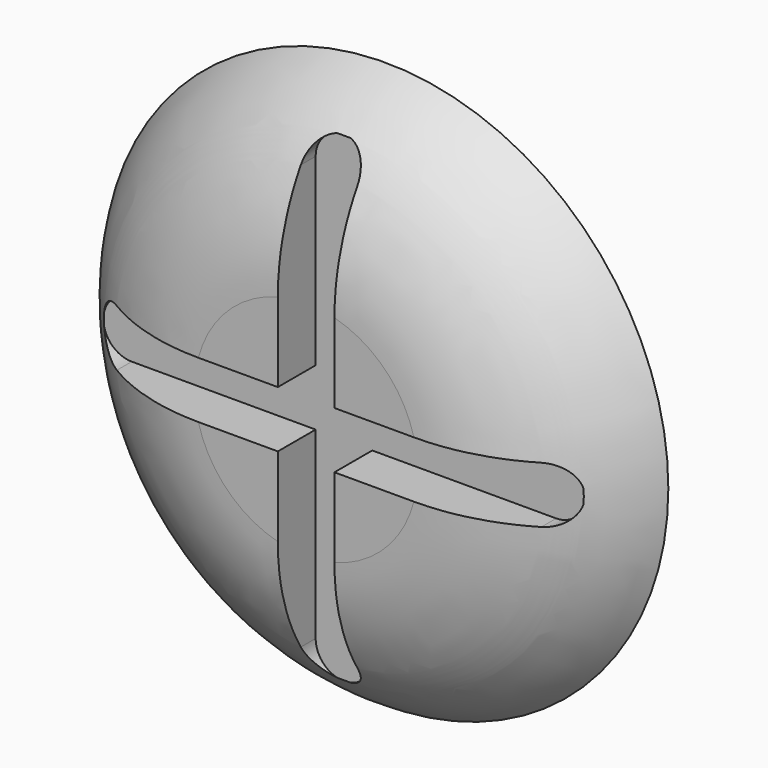
from build123d import *

# Parameters (mm, degrees)
F0_R     = 25.4
F1_DEPTH = 8.89
F3_W     = 5.08
F3_H     = 5.08
F4_DEPTH = 4.2418


# Not quite as in the source:
# - a fillet or chamfer that OpenCascade refuses, or shapes differently, is made with other operations: its cross-section is extruded or revolved along the edge and cut away or added


with BuildPart() as f1:
    # F0 (on Front) → F1 (new body)
    with BuildSketch(Plane.XZ):
        Circle(F0_R)
    extrude(amount=F1_DEPTH)

    # F2: fillet of radius 17.7830971004 on 1 edges, made by hand

    # F2_s1 → F2_t2 (revolve, cut)
    with BuildSketch(Plane.XY):
        with BuildLine():
            ThreePointArc((25.4, 0), (18.8910545541, -6.507963768), (10.0002803128, -8.89))
            Line((10.0002803128, -8.89), (25.4, -8.89))
            Line((25.4, -8.89), (25.4, 0))
        make_face()
    revolve(axis=Axis((0, -8.89, 0), (0, -1, 0)), mode=Mode.SUBTRACT)

    # F3 (on face) → F4 (cut)
    with BuildSketch(Plane.XZ.offset(8.89)):
        with BuildLine():
            Line((2.54, 19.05), (-2.54, 19.05))
            Line((-2.54, 19.05), (-2.54, 9.6723320008))
            ThreePointArc((-2.54, 9.6723320008), (0, 10.0002803128), (2.54, 9.6723320008))
            Line((2.54, 9.6723320008), (2.54, 19.05))
        make_face()
        with BuildLine():
            ThreePointArc((2.54, 19.05), (0, 21.59), (-2.54, 19.05))
            Line((-2.54, 19.05), (2.54, 19.05))
        make_face()
        with BuildLine():
            ThreePointArc((2.54, 9.6723320008), (0, 10.0002803128), (-2.54, 9.6723320008))
            Line((-2.54, 9.6723320008), (-2.54, 2.54))
            Line((-2.54, 2.54), (2.54, 2.54))
            Line((2.54, 2.54), (2.54, 9.6723320008))
        make_face()
        Rectangle(F3_W, F3_H)
        with BuildLine():
            Line((2.54, -2.54), (-2.54, -2.54))
            Line((-2.54, -2.54), (-2.54, -9.6723320008))
            ThreePointArc((-2.54, -9.6723320008), (0, -10.0002803128), (2.54, -9.6723320008))
            Line((2.54, -9.6723320008), (2.54, -2.54))
        make_face()
        with BuildLine():
            Line((2.54, -19.05), (-2.54, -19.05))
            ThreePointArc((-2.54, -19.05), (0, -21.59), (2.54, -19.05))
        make_face()
        with BuildLine():
            ThreePointArc((2.54, -9.6723320008), (0, -10.0002803128), (-2.54, -9.6723320008))
            Line((-2.54, -9.6723320008), (-2.54, -19.05))
            Line((-2.54, -19.05), (2.54, -19.05))
            Line((2.54, -19.05), (2.54, -9.6723320008))
        make_face()
        with BuildLine():
            Line((9.6723320008, 2.54), (2.54, 2.54))
            Line((2.54, 2.54), (2.54, -2.54))
            Line((2.54, -2.54), (9.6723320008, -2.54))
            ThreePointArc((9.6723320008, -2.54), (9.9179543662, -1.2805418868), (10.0002803128, 0))
            ThreePointArc((10.0002803128, 0), (9.9179543662, 1.2805418868), (9.6723320008, 2.54))
        make_face()
        with BuildLine():
            Line((19.05, 2.54), (9.6723320008, 2.54))
            ThreePointArc((9.6723320008, 2.54), (9.9179543662, 1.2805418868), (10.0002803128, 0))
            ThreePointArc((10.0002803128, 0), (9.9179543662, -1.2805418868), (9.6723320008, -2.54))
            Line((9.6723320008, -2.54), (19.05, -2.54))
            Line((19.05, -2.54), (19.05, 2.54))
        make_face()
        with BuildLine():
            ThreePointArc((19.05, -2.54), (21.59, 0), (19.05, 2.54))
            Line((19.05, 2.54), (19.05, -2.54))
        make_face()
        with BuildLine():
            Line((-2.54, -2.54), (-2.54, 2.54))
            Line((-2.54, 2.54), (-9.6723320008, 2.54))
            ThreePointArc((-9.6723320008, 2.54), (-10.0002803128, 0), (-9.6723320008, -2.54))
            Line((-9.6723320008, -2.54), (-2.54, -2.54))
        make_face()
        with BuildLine():
            ThreePointArc((-9.6723320008, -2.54), (-10.0002803128, 0), (-9.6723320008, 2.54))
            Line((-9.6723320008, 2.54), (-19.05, 2.54))
            Line((-19.05, 2.54), (-19.05, -2.54))
            Line((-19.05, -2.54), (-9.6723320008, -2.54))
        make_face()
        with BuildLine():
            Line((-19.05, -2.54), (-19.05, 2.54))
            ThreePointArc((-19.05, 2.54), (-21.59, 0), (-19.05, -2.54))
        make_face()
    extrude(amount=-F4_DEPTH, mode=Mode.SUBTRACT)


solid = f1.part
